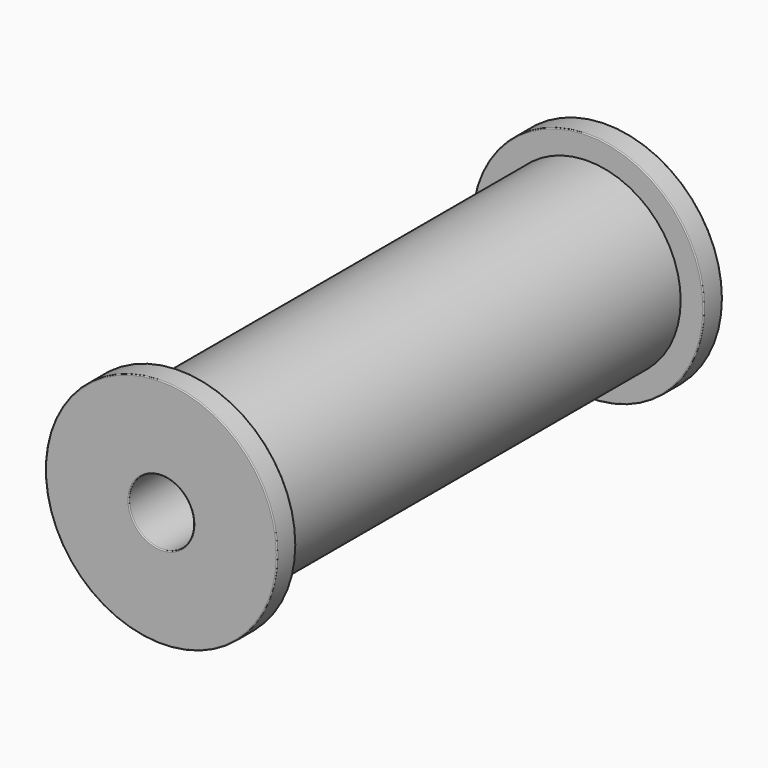
from build123d import *

# Parameters (mm, degrees)
F0_R     = 25
F1_DEPTH = 5
F2_R     = 20
F3_DEPTH = 110
F5_R     = 25
F4_R     = 20
F6_DEPTH = 5
F7_R     = 7
F8_DEPTH = 200
F9_R     = 0.2


# Not quite as in the source:
# - a feature names something its author has since deleted; it is built from what else it names


with BuildPart() as f1:
    # F0 (on Front) → F1 (new body)
    with BuildSketch(Plane.XZ):
        Circle(F0_R)
    extrude(amount=F1_DEPTH)

    # F2 (on face) → F3 (join)
    with BuildSketch(Plane.XZ.offset(5)):
        Circle(F2_R)
    extrude(amount=F3_DEPTH)

    # F5 (on face) + F4 (on face) → F6 (join)
    with BuildSketch(Plane.XZ.offset(115)):
        Circle(F5_R)
    with BuildSketch(Plane.XZ.offset(115)):
        Circle(F4_R)
    extrude(amount=F6_DEPTH)

    # F7 (on face) → F8 (cut)
    with BuildSketch(Plane.XZ.offset(120)):
        Circle(F7_R)
    extrude(amount=-F8_DEPTH, mode=Mode.SUBTRACT)

    # F9
    f9_edges = [f1.edges().sort_by_distance(p)[0] for p in [
        (-25, -120, 0),
        (-7, -120, 0),
        (-25, -115, 0),
        (-25, -5, 0),
        (-25, 0, 0),
        (-7, 0, 0),
    ]]
    fillet(f9_edges, radius=F9_R)


solid = f1.part
